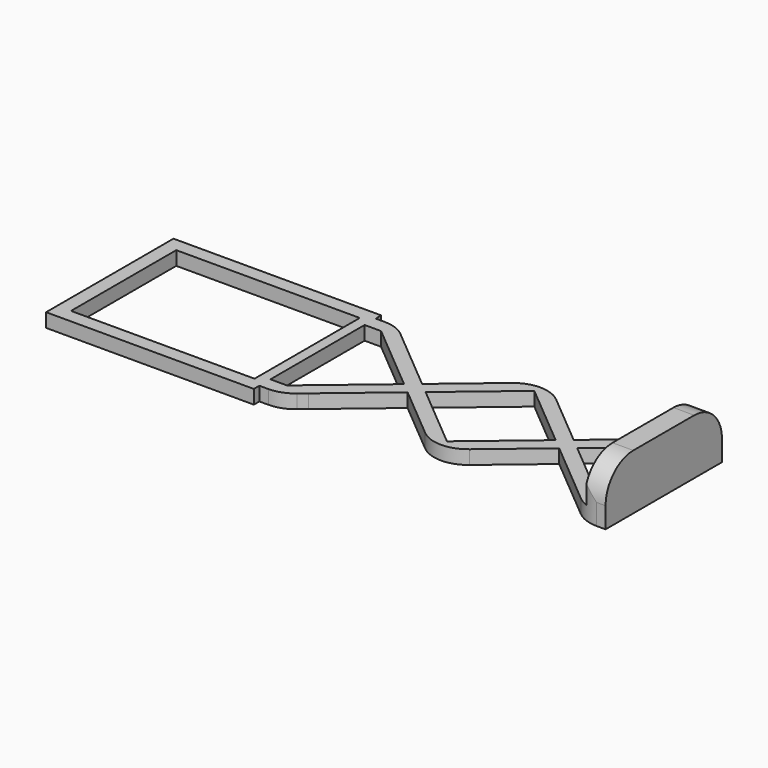
from build123d import *

# Parameters (mm, degrees)
F0_W        = 26.5
F0_H        = 19
F1_DEPTH    = 2
F2_DEPTH    = 8
F3_T1_DEPTH = 23
F3_T3_DEPTH = 11.1067326603
F3_T5_DEPTH = 28


# Not quite as in the source:
# - a fillet or chamfer that OpenCascade refuses, or shapes differently, is made with other operations: its cross-section is extruded or revolved along the edge and cut away or added


with BuildPart() as f1:
    # F0 (on Top) → F1 (new body)
    with BuildSketch(Plane.XY):
        Polygon((-5.2328903973, 8.0285165012), (-35.2328903973, 8.0285165012), (-35.2328903973, -14.9714834988), (-5.2328903973, -14.9714834988), (-5.2328903973, -13.9714834988), (-5.2328903973, -11.9714834988), (-5.2328903973, 5.0285165012), (-5.2328903973, 7.0285165012), align=None)
        with Locations((-19.9828903973, -3.4714834988)):
            Rectangle(F0_W, F0_H, mode=Mode.SUBTRACT)
        Polygon((-2.8519380164, 5.0285165012), (-5.2328903973, 7.0285165012), (-5.2328903973, 5.0285165012), align=None)
        Polygon((-2.1233994035, 7.0285165012), (-5.2328903973, 7.0285165012), (-2.8519380164, 5.0285165012), (0.2575529774, 5.0285165012), align=None)
        Polygon((0.2575529774, 5.0285165012), (-2.8519380164, 5.0285165012), (7.2671096027, -3.4714834988), (8.8218550996, -2.1654972814), align=None)
        Polygon((-5.2328903973, -11.9714834988), (-5.2328903973, -13.9714834988), (-2.8519380164, -11.9714834988), align=None)
        Polygon((-2.8519380164, -11.9714834988), (-5.2328903973, -13.9714834988), (-2.1233994035, -13.9714834988), (0.2575529774, -11.9714834988), align=None)
        Polygon((8.8218550996, -4.7774697162), (7.2671096027, -3.4714834988), (-2.8519380164, -11.9714834988), (0.2575529774, -11.9714834988), align=None)
        Polygon((8.8218550996, -2.1654972814), (7.2671096027, -3.4714834988), (8.8218550996, -4.7774697162), (10.3766005965, -3.4714834988), align=None)
        Polygon((21.3218550996, 5.7225302838), (19.7671096027, 7.0285165012), (8.8218550996, -2.1654972814), (10.3766005965, -3.4714834988), (19.7671096027, 4.4165440664), align=None)
        Polygon((10.3766005965, -3.4714834988), (8.8218550996, -4.7774697162), (19.7671096027, -13.9714834988), (21.3218550996, -12.6654972814), (19.7671096027, -11.359511064), align=None)
        Polygon((19.7671096027, -11.359511064), (21.3218550996, -12.6654972814), (30.7123641058, -4.7774697162), (29.1576186089, -3.4714834988), align=None)
        Polygon((30.7123641058, -2.1654972814), (21.3218550996, 5.7225302838), (19.7671096027, 4.4165440664), (29.1576186089, -3.4714834988), align=None)
        Polygon((32.2671096027, -3.4714834988), (30.7123641058, -2.1654972814), (29.1576186089, -3.4714834988), (30.7123641058, -4.7774697162), align=None)
        Polygon((41.7671096027, 7.0285165012), (41.6576186089, 7.0285165012), (30.7123641058, -2.1654972814), (32.2671096027, -3.4714834988), (41.7671096027, 4.5085165012), align=None)
        Polygon((30.7123641058, -4.7774697162), (41.6576186089, -13.9714834988), (41.7671096027, -13.9714834988), (41.7671096027, -11.4514834988), (32.2671096027, -3.4714834988), align=None)
    extrude(amount=F1_DEPTH)

    # F0 (on Top) → F2 (join)
    with BuildSketch(Plane.XY):
        Polygon((44.7671096027, 7.0285165012), (41.7671096027, 7.0285165012), (41.7671096027, 4.5085165012), align=None)
        Polygon((44.7671096027, 7.0285165012), (41.7671096027, 4.5085165012), (41.7671096027, -11.4514834988), (44.7671096027, -13.9714834988), align=None)
        Polygon((41.7671096027, -11.4514834988), (41.7671096027, -13.9714834988), (44.7671096027, -13.9714834988), align=None)
    extrude(amount=F2_DEPTH)

    # F3: fillet of radius 5 on 8 edges, made by hand

    # F3_s2 → F3_t1 (cut)
    with BuildSketch(Plane.XY.offset(-10.5)):
        with BuildLine():
            ThreePointArc((22.9830700348, -11.2700767358), (19.7671096027, -12.4415524119), (16.5511491706, -11.2700767358))
            Line((16.5511491706, -11.2700767358), (19.7671096027, -13.9714834988))
            Line((19.7671096027, -13.9714834988), (22.9830700348, -11.2700767358))
        make_face()
        with BuildLine():
            ThreePointArc((16.5511491706, 4.3271097382), (19.7671096027, 5.4985854143), (22.9830700348, 4.3271097382))
            Line((22.9830700348, 4.3271097382), (19.7671096027, 7.0285165012))
            Line((19.7671096027, 7.0285165012), (16.5511491706, 4.3271097382))
        make_face()
    extrude(amount=F3_T1_DEPTH, mode=Mode.SUBTRACT)

    # F3_s4 → F3_t3 (cut)
    with BuildSketch(Plane.XY.offset(-4.5533663301)):
        with BuildLine():
            ThreePointArc((-0.7287855035, -12.8000078228), (-2.2334045932, -13.6694948664), (-3.9447459356, -13.9714834988))
            Line((-3.9447459356, -13.9714834988), (-2.1233994035, -13.9714834988))
            Line((-2.1233994035, -13.9714834988), (-0.7287855035, -12.8000078228))
        make_face()
        with BuildLine():
            ThreePointArc((-3.9447459356, 7.0285165012), (-2.2334045932, 6.7265278688), (-0.7287855035, 5.8570408251))
            Line((-0.7287855035, 5.8570408251), (-2.1233994035, 7.0285165012))
            Line((-2.1233994035, 7.0285165012), (-3.9447459356, 7.0285165012))
        make_face()
        with BuildLine():
            ThreePointArc((40.2630047089, 5.8570408251), (41.7676237986, 6.7265278688), (43.478965141, 7.0285165012))
            Line((43.478965141, 7.0285165012), (41.6576186089, 7.0285165012))
            Line((41.6576186089, 7.0285165012), (40.2630047089, 5.8570408251))
        make_face()
        with BuildLine():
            ThreePointArc((43.478965141, -13.9714834988), (41.7676237986, -13.6694948664), (40.2630047089, -12.8000078228))
            Line((40.2630047089, -12.8000078228), (41.6576186089, -13.9714834988))
            Line((41.6576186089, -13.9714834988), (43.478965141, -13.9714834988))
        make_face()
    extrude(amount=F3_T3_DEPTH, mode=Mode.SUBTRACT)

    # F3_s6 → F3_t5 (cut)
    with BuildSketch(Plane.YZ.offset(29.2671096027)):
        with BuildLine():
            ThreePointArc((-8.9714834988, 8), (-12.5070174047, 6.5355339059), (-13.9714834988, 3))
            Line((-13.9714834988, 3), (-13.9714834988, 8))
            Line((-13.9714834988, 8), (-8.9714834988, 8))
        make_face()
        with BuildLine():
            ThreePointArc((7.0285165012, 3), (5.5640504071, 6.5355339059), (2.0285165012, 8))
            Line((2.0285165012, 8), (7.0285165012, 8))
            Line((7.0285165012, 8), (7.0285165012, 3))
        make_face()
    extrude(amount=F3_T5_DEPTH, mode=Mode.SUBTRACT)


solid = f1.part
